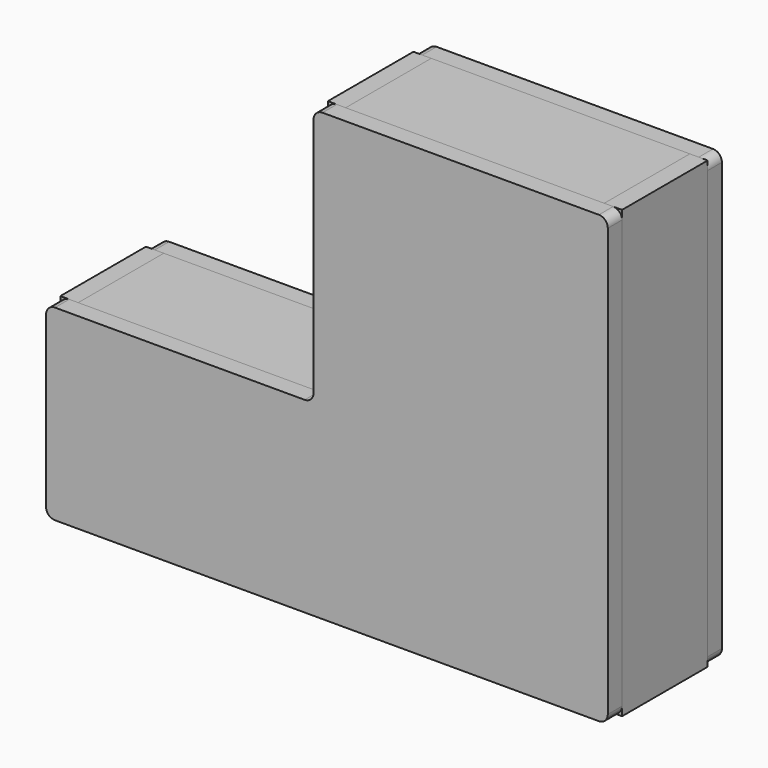
from build123d import *

# Parameters (mm, degrees)
F1_DEPTH     = 10
F3_DEPTH     = 60
F2_W         = 140
F2_H         = 10
F4_DEPTH     = 60
F5_DEPTH     = 60
F2_W_2       = 145
F6_DEPTH     = 60
F7_DEPTH     = 60
F2_W_3       = 295
F8_DEPTH     = 60
F10_DEPTH    = 13
F12_DEPTH    = 10
F13_R        = 5
F14_R        = 5
F14_2_R      = 5
F15_W        = 60
F15_H        = 10
F16_DEPTH    = 20
F17_W        = 60
F17_H        = 10
F18_DEPTH    = 20
F20_D        = 4
F23_D        = 3.5
F23_ON_F22_D = 3.5


with BuildPart() as f1:
    # F0 (on Front) → F1 (new body)
    with BuildSketch(Plane.XZ):
        Polygon((-267.2632135372, 120.211422946), (-432.2632135372, 120.211422946), (-432.2632135372, -24.788577054), (-582.2632135372, -24.788577054), (-582.2632135372, -129.788577054), (-267.2632135372, -129.788577054), align=None)
    extrude(amount=F1_DEPTH)

    # F14
    f14_edges = [f1.edges().sort_by_distance(p)[0] for p in [
        (-582.263214, -5, -129.788577),
        (-582.263214, -5, -24.788577),
        (-432.263214, -5, -24.788577),
        (-432.263214, -5, 120.211423),
        (-267.263214, -5, 120.211423),
        (-267.263214, -5, -129.788577),
    ]]
    fillet(f14_edges, radius=F14_R)


with BuildPart() as f3:
    # F2 (on face) → F3 (new body)
    with BuildSketch(Plane.XZ.offset(10)):
        Polygon((-572.2632135372, -24.788577054), (-582.2632135372, -24.788577054), (-582.2632135372, -129.788577054), (-572.2632135372, -129.788577054), (-572.2632135372, -119.788577054), (-572.2632135372, -34.788577054), align=None)
    extrude(amount=F3_DEPTH)


with BuildPart() as f4:
    # F2 (on face) → F4 (new body)
    with BuildSketch(Plane.XZ.offset(10)):
        with Locations((-502.2632135372, -29.788577054)):
            Rectangle(F2_W, F2_H)
    extrude(amount=F4_DEPTH)


with BuildPart() as f5:
    # F2 (on face) → F5 (new body)
    with BuildSketch(Plane.XZ.offset(10)):
        Polygon((-432.2632135372, 120.211422946), (-432.2632135372, -24.788577054), (-432.2632135372, -34.788577054), (-422.2632135372, -34.788577054), (-422.2632135372, 110.211422946), (-422.2632135372, 120.211422946), align=None)
    extrude(amount=F5_DEPTH)


with BuildPart() as f6:
    # F2 (on face) → F6 (new body)
    with BuildSketch(Plane.XZ.offset(10)):
        with Locations((-349.7632135372, 115.211422946)):
            Rectangle(F2_W_2, F2_H)
    extrude(amount=F6_DEPTH)


with BuildPart() as f7:
    # F2 (on face) → F7 (new body)
    with BuildSketch(Plane.XZ.offset(10)):
        Polygon((-277.2632135372, -119.788577054), (-277.2632135372, -129.788577054), (-267.2632135372, -129.788577054), (-267.2632135372, 120.211422946), (-277.2632135372, 120.211422946), (-277.2632135372, 110.211422946), align=None)
    extrude(amount=F7_DEPTH)


with BuildPart() as f8:
    # F2 (on face) → F8 (new body)
    with BuildSketch(Plane.XZ.offset(10)):
        with Locations((-424.7632135372, -124.788577054)):
            Rectangle(F2_W_3, F2_H)
    extrude(amount=F8_DEPTH)

    # F9 (on face) → F10 (cut)
    with BuildSketch(Plane(origin=(0, 0, -129.788577054), x_dir=(1, 0, 0), z_dir=(0, 0, -1))):
        with BuildLine():
            Line((-512.2632135372, 55), (-532.2632135372, 55))
            ThreePointArc((-532.2632135372, 55), (-535.7987474431, 53.5355339059), (-537.2632135372, 50))
            Line((-537.2632135372, 50), (-537.2632135372, 30))
            ThreePointArc((-537.2632135372, 30), (-535.7987474431, 26.4644660941), (-532.2632135372, 25))
            Line((-532.2632135372, 25), (-512.2632135372, 25))
            ThreePointArc((-512.2632135372, 25), (-508.7276796312, 26.4644660941), (-507.2632135372, 30))
            Line((-507.2632135372, 30), (-507.2632135372, 50))
            ThreePointArc((-507.2632135372, 50), (-508.7276796312, 53.5355339059), (-512.2632135372, 55))
        make_face()
        with BuildLine():
            Line((-317.2632135372, 55), (-337.2632135372, 55))
            ThreePointArc((-337.2632135372, 55), (-340.7987474431, 53.5355339059), (-342.2632135372, 50))
            Line((-342.2632135372, 50), (-342.2632135372, 30))
            ThreePointArc((-342.2632135372, 30), (-340.7987474431, 26.4644660941), (-337.2632135372, 25))
            Line((-337.2632135372, 25), (-317.2632135372, 25))
            ThreePointArc((-317.2632135372, 25), (-313.7276796312, 26.4644660941), (-312.2632135372, 30))
            Line((-312.2632135372, 30), (-312.2632135372, 50))
            ThreePointArc((-312.2632135372, 50), (-313.7276796312, 53.5355339059), (-317.2632135372, 55))
        make_face()
    extrude(amount=-F10_DEPTH, mode=Mode.SUBTRACT)

    # F20 (through all)
    with Locations(Plane(origin=(0, 0, -129.788577054), x_dir=(1, 0, 0), z_dir=(0, 0, -1))):
        with Locations((-562.2632135372, 55), (-562.2632135372, 25), (-287.2632135372, 55), (-287.2632135372, 25)):
            Hole(F20_D / 2)


with BuildPart() as f12:
    # F11 (on face) → F12 (new body)
    with BuildSketch(Plane.XZ.offset(70)):
        Polygon((-267.2632135372, 120.211422946), (-432.2632135372, 120.211422946), (-432.2632135372, -24.788577054), (-582.2632135372, -24.788577054), (-582.2632135372, -129.788577054), (-267.2632135372, -129.788577054), align=None)
    extrude(amount=F12_DEPTH)

    # F13
    f13_edges = [f12.edges().sort_by_distance(p)[0] for p in [
        (-582.263214, -75, -129.788577),
    ]]
    fillet(f13_edges, radius=F13_R)

    # F14#2
    f14_2_edges = [f12.edges().sort_by_distance(p)[0] for p in [
        (-582.263214, -75, -24.788577),
        (-432.263214, -75, -24.788577),
        (-432.263214, -75, 120.211423),
        (-267.263214, -75, 120.211423),
        (-267.263214, -75, -129.788577),
    ]]
    fillet(f14_2_edges, radius=F14_2_R)


with BuildPart() as f16:
    # F15 (on face) → F16 (new body)
    with BuildSketch(Plane.YZ.offset(-572.2632135372)):
        with Locations((-40, -114.788577054)):
            Rectangle(F15_W, F15_H)
    extrude(amount=F16_DEPTH)

    # F23 (through all)
    with Locations(Plane(origin=(0, 0, -119.788577054), x_dir=(1, 0, 0), z_dir=(0, 0, -1))):
        with Locations((-562.2632135372, 55), (-562.2632135372, 25)):
            Hole(F23_D / 2)


with BuildPart() as f18:
    # F17 (on face) → F18 (new body)
    with BuildSketch(Plane(origin=(-277.2632135372, 0, 0), x_dir=(0, -1, 0), z_dir=(-1, 0, 0))):
        with Locations((40, -114.788577054)):
            Rectangle(F17_W, F17_H)
    extrude(amount=F18_DEPTH)

    # F23 on F22 (through all)
    with Locations(Plane(origin=(0, 0, -119.788577054), x_dir=(1, 0, 0), z_dir=(0, 0, -1))):
        with Locations((-287.2632135372, 55), (-287.2632135372, 25)):
            Hole(F23_ON_F22_D / 2)


solid = Compound([f1.part, f3.part, f4.part, f5.part, f6.part, f7.part, f8.part, f12.part, f16.part, f18.part])
